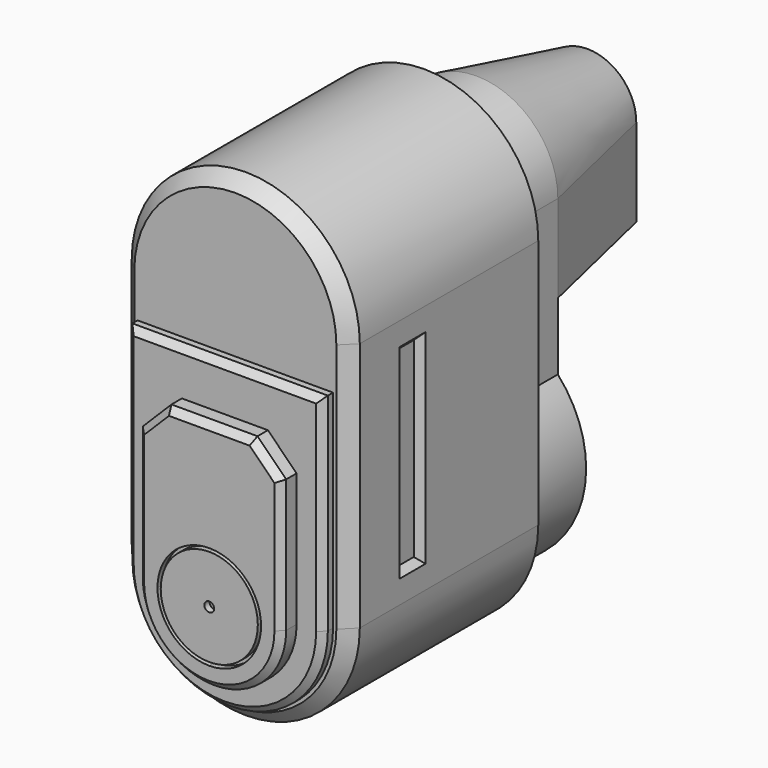
from build123d import *

# Parameters (mm, degrees)
F1_DEPTH  = 36.232
F2_DEPTH  = 2
F4_DEPTH  = 3
F5_SIZE   = 1
F6_SIZE   = 4.4
F7_SIZE   = 1
F8_R      = 0.75
F9_DEPTH  = 1
F10_SIZE  = 2
F11_W     = 5
F11_H     = 31.3
F12_DEPTH = 1
F13_W     = 5
F13_H     = 31.3
F14_DEPTH = 1
F15_SIZE  = 0.99999
F17_DEPTH = 10
F18_DEPTH = 1


# Not quite as in the source:
# - a fillet or chamfer is up to 0.001 mm smaller than in the source, because OpenCascade refuses the exact size


with BuildPart() as f1:
    # F0 (on Front) → F1 (new body)
    with BuildSketch(Plane.XZ):
        with BuildLine():
            Line((-17.5, 38.4), (-17.5, 0))
            ThreePointArc((-17.5, 0), (0, -17.5), (17.5, 0))
            Line((17.5, 0), (17.5, 38.4))
            ThreePointArc((17.5, 38.4), (0, 55.9), (-17.5, 38.4))
        make_face()
        with BuildLine():
            ThreePointArc((15, 0), (0, -15), (-15, 0))
            Line((-15, 0), (-15, 31.8))
            Line((-15, 31.8), (-15, 38.4))
            ThreePointArc((-15, 38.4), (0, 53.4), (15, 38.4))
            Line((15, 38.4), (15, 31.8))
            Line((15, 31.8), (15, 0))
        make_face(mode=Mode.SUBTRACT)
        with BuildLine():
            Line((-15, 31.8), (-15, 0))
            ThreePointArc((-15, 0), (0, -15), (15, 0))
            Line((15, 0), (15, 31.8))
            Line((15, 31.8), (-15, 31.8))
        make_face()
        with BuildLine():
            ThreePointArc((11, 0), (0, -11), (-11, 0))
            Line((-11, 0), (-11, 24.8))
            Line((-11, 24.8), (11, 24.8))
            Line((11, 24.8), (11, 0))
        make_face(mode=Mode.SUBTRACT)
        with BuildLine():
            Line((-11, 24.8), (-11, 0))
            ThreePointArc((-11, 0), (0, -11), (11, 0))
            Line((11, 0), (11, 24.8))
            Line((11, 24.8), (-11, 24.8))
        make_face()
        with BuildLine():
            ThreePointArc((0, -7.95), (-5.6214989104, -5.6214989104), (-7.95, 0))
            ThreePointArc((-7.95, 0), (-5.6214989104, 5.6214989104), (0, 7.95))
            ThreePointArc((0, 7.95), (5.6214989104, 5.6214989104), (7.95, 0))
            ThreePointArc((7.95, 0), (5.6214989104, -5.6214989104), (0, -7.95))
        make_face(mode=Mode.SUBTRACT)
        with BuildLine():
            Line((-15, 38.4), (-15, 31.8))
            Line((-15, 31.8), (15, 31.8))
            Line((15, 31.8), (15, 38.4))
            ThreePointArc((15, 38.4), (0, 53.4), (-15, 38.4))
        make_face()
        with BuildLine():
            ThreePointArc((0, 7.95), (-5.6214989104, 5.6214989104), (-7.95, 0))
            ThreePointArc((-7.95, 0), (-5.6214989104, -5.6214989104), (0, -7.95))
            ThreePointArc((0, -7.95), (5.6214989104, -5.6214989104), (7.95, 0))
            ThreePointArc((7.95, 0), (5.6214989104, 5.6214989104), (0, 7.95))
        make_face()
    extrude(amount=-F1_DEPTH)

    # F10
    f10_edges = [f1.edges().sort_by_distance(p)[0] for p in [
        (-17.5, 0, 19.2),
    ]]
    chamfer(f10_edges, length=F10_SIZE)

    # F11 (on face) → F12 (cut)
    with BuildSketch(Plane(origin=(-17.5, 0, 0), x_dir=(0, -1, 0), z_dir=(-1, 0, 0))):
        with Locations((-12.1, 19.2)):
            Rectangle(F11_W, F11_H)
    extrude(amount=-F12_DEPTH, mode=Mode.SUBTRACT)

    # F13 (on face) → F14 (cut)
    with BuildSketch(Plane.YZ.offset(17.5)):
        with Locations((12.1, 19.2)):
            Rectangle(F13_W, F13_H)
    extrude(amount=-F14_DEPTH, mode=Mode.SUBTRACT)

    # F15 (size 1 in the source; OpenCascade refuses exactly that, so slightly less here)
    f15_edges = [f1.edges().sort_by_distance(p)[0] for p in [
        (16.5, 14.6, 19.2),
        (16.5, 9.6, 19.2),
        (16.5, 12.1, 34.85),
        (16.5, 12.1, 3.55),
        (-16.5, 12.1, 3.55),
        (-16.5, 9.6, 19.2),
        (-16.5, 12.1, 34.85),
        (-16.5, 14.6, 19.2),
    ]]
    chamfer(f15_edges, length=F15_SIZE)

    # F16 (on face) → F17 (join)
    with BuildSketch(Plane(origin=(0, 36.232, 0), x_dir=(-1, 0, 0), z_dir=(0, 1, 0))):
        with BuildLine():
            ThreePointArc((12.5, 38.4), (0, 50.9), (-12.5, 38.4))
            Line((-12.5, 38.4), (-12.5, 14.6492256372))
            ThreePointArc((-12.5, 14.6492256372), (0, -13.5), (12.5, 14.6492256372))
            Line((12.5, 14.6492256372), (12.5, 38.4))
        make_face()
        with BuildLine():
            ThreePointArc((-11.5, 38.4), (0, 49.9), (11.5, 38.4))
            Line((11.5, 38.4), (11.5, 14.2574515814))
            ThreePointArc((11.5, 14.2574515814), (0, -12.5), (-11.5, 14.2574515814))
            Line((-11.5, 14.2574515814), (-11.5, 38.4))
        make_face(mode=Mode.SUBTRACT)
    extrude(amount=F17_DEPTH)

    # F16 (on face) → F18 (cut)
    with BuildSketch(Plane(origin=(0, 36.232, 0), x_dir=(-1, 0, 0), z_dir=(0, 1, 0))):
        with BuildLine():
            ThreePointArc((0, -7.95), (5.6214989104, -5.6214989104), (7.95, 0))
            ThreePointArc((7.95, 0), (5.6214989104, 5.6214989104), (0, 7.95))
            ThreePointArc((0, 7.95), (-5.6214989104, 5.6214989104), (-7.95, 0))
            ThreePointArc((-7.95, 0), (-5.6214989104, -5.6214989104), (0, -7.95))
        make_face()
    extrude(amount=-F18_DEPTH, mode=Mode.SUBTRACT)

    # F19 (on face) → F22 section 0
    with BuildSketch(Plane(origin=(0, 46.232, 0), x_dir=(-1, 0, 0), z_dir=(0, 1, 0))):
        with BuildLine():
            Line((12.5, 24.958), (12.5, 38.4))
            ThreePointArc((12.5, 38.4), (0, 50.9), (-12.5, 38.4))
            Line((-12.5, 38.4), (-12.5, 24.958))
            Line((-12.5, 24.958), (-11.5, 24.958))
            Line((-11.5, 24.958), (-11.5, 38.4))
            ThreePointArc((-11.5, 38.4), (0, 49.9), (11.5, 38.4))
            Line((11.5, 38.4), (11.5, 24.958))
            Line((11.5, 24.958), (12.5, 24.958))
        make_face()
    # F21 (on offset) → F22 section 1
    with BuildSketch(Plane(origin=(0, 67.532, 0), x_dir=(-1, 0, 0), z_dir=(0, 1, 0))):
        with BuildLine():
            ThreePointArc((7.5, 38.4), (0, 45.9), (-7.5, 38.4))
            Line((-7.5, 38.4), (-7.5, 24.958))
            Line((-7.5, 24.958), (-6.5, 24.958))
            Line((-6.5, 24.958), (-6.5, 38.4))
            ThreePointArc((-6.5, 38.4), (0, 44.9), (6.5, 38.4))
            Line((6.5, 38.4), (6.5, 24.958))
            Line((6.5, 24.958), (7.5, 24.958))
            Line((7.5, 24.958), (7.5, 38.4))
        make_face()
    loft()


with BuildPart() as f2:
    # F0 (on Front) → F2 (new body)
    with BuildSketch(Plane.XZ):
        with BuildLine():
            Line((-15, 31.8), (-15, 0))
            ThreePointArc((-15, 0), (0, -15), (15, 0))
            Line((15, 0), (15, 31.8))
            Line((15, 31.8), (-15, 31.8))
        make_face()
        with BuildLine():
            ThreePointArc((11, 0), (0, -11), (-11, 0))
            Line((-11, 0), (-11, 24.8))
            Line((-11, 24.8), (11, 24.8))
            Line((11, 24.8), (11, 0))
        make_face(mode=Mode.SUBTRACT)
        with BuildLine():
            Line((-11, 24.8), (-11, 0))
            ThreePointArc((-11, 0), (0, -11), (11, 0))
            Line((11, 0), (11, 24.8))
            Line((11, 24.8), (-11, 24.8))
        make_face()
        with BuildLine():
            ThreePointArc((0, -7.95), (-5.6214989104, -5.6214989104), (-7.95, 0))
            ThreePointArc((-7.95, 0), (-5.6214989104, 5.6214989104), (0, 7.95))
            ThreePointArc((0, 7.95), (5.6214989104, 5.6214989104), (7.95, 0))
            ThreePointArc((7.95, 0), (5.6214989104, -5.6214989104), (0, -7.95))
        make_face(mode=Mode.SUBTRACT)
        with BuildLine():
            ThreePointArc((0, 7.95), (-5.6214989104, 5.6214989104), (-7.95, 0))
            ThreePointArc((-7.95, 0), (-5.6214989104, -5.6214989104), (0, -7.95))
            ThreePointArc((0, -7.95), (5.6214989104, -5.6214989104), (7.95, 0))
            ThreePointArc((7.95, 0), (5.6214989104, 5.6214989104), (0, 7.95))
        make_face()
    extrude(amount=F2_DEPTH)

    # F3 (on face) → F4 (join)
    with BuildSketch(Plane.XZ.offset(2)):
        with BuildLine():
            Line((-11, 24.8), (-11, 0))
            ThreePointArc((-11, 0), (0, -11), (11, 0))
            Line((11, 0), (11, 24.8))
            Line((11, 24.8), (-11, 24.8))
        make_face()
        with BuildLine():
            ThreePointArc((0, 7.95), (5.6214989104, 5.6214989104), (7.95, 0))
            ThreePointArc((7.95, 0), (5.6214989104, -5.6214989104), (0, -7.95))
            ThreePointArc((0, -7.95), (-5.6214989104, -5.6214989104), (-7.95, 0))
            ThreePointArc((-7.95, 0), (-5.6214989104, 5.6214989104), (0, 7.95))
        make_face(mode=Mode.SUBTRACT)
        with BuildLine():
            ThreePointArc((0, -7.95), (5.6214989104, -5.6214989104), (7.95, 0))
            ThreePointArc((7.95, 0), (5.6214989104, 5.6214989104), (0, 7.95))
            ThreePointArc((0, 7.95), (-5.6214989104, 5.6214989104), (-7.95, 0))
            ThreePointArc((-7.95, 0), (-5.6214989104, -5.6214989104), (0, -7.95))
        make_face()
    extrude(amount=F4_DEPTH)

    # F5
    f5_edges = [f2.edges().sort_by_distance(p)[0] for p in [
        (0, -2, 31.8),
        (-15, -2, 15.9),
    ]]
    chamfer(f5_edges, length=F5_SIZE)

    # F6
    f6_edges = [f2.edges().sort_by_distance(p)[0] for p in [
        (11, -3.5, 24.8),
        (-11, -3.5, 24.8),
    ]]
    chamfer(f6_edges, length=F6_SIZE)

    # F7
    f7_edges = [f2.edges().sort_by_distance(p)[0] for p in [
        (-11, -5, 10.2),
        (0, -5, 24.8),
        (-8.8, -5, 22.6),
        (8.8, -5, 22.6),
    ]]
    chamfer(f7_edges, length=F7_SIZE)

    # F8 (on face) → F9 (cut)
    with BuildSketch(Plane.XZ.offset(5)):
        with BuildLine():
            ThreePointArc((0, 7.95), (-5.6214989104, 5.6214989104), (-7.95, 0))
            ThreePointArc((-7.95, 0), (-5.6214989104, -5.6214989104), (0, -7.95))
            ThreePointArc((0, -7.95), (5.6214989104, -5.6214989104), (7.95, 0))
            ThreePointArc((7.95, 0), (5.6214989104, 5.6214989104), (0, 7.95))
        make_face()
        with BuildLine():
            ThreePointArc((0, -7.45), (-5.2679455198, -5.2679455198), (-7.45, 0))
            ThreePointArc((-7.45, 0), (-5.2679455198, 5.2679455198), (0, 7.45))
            ThreePointArc((0, 7.45), (5.2679455198, 5.2679455198), (7.45, 0))
            ThreePointArc((7.45, 0), (5.2679455198, -5.2679455198), (0, -7.45))
        make_face(mode=Mode.SUBTRACT)
        Circle(F8_R)
    extrude(amount=-F9_DEPTH, mode=Mode.SUBTRACT)


solid = Compound([f1.part, f2.part])
